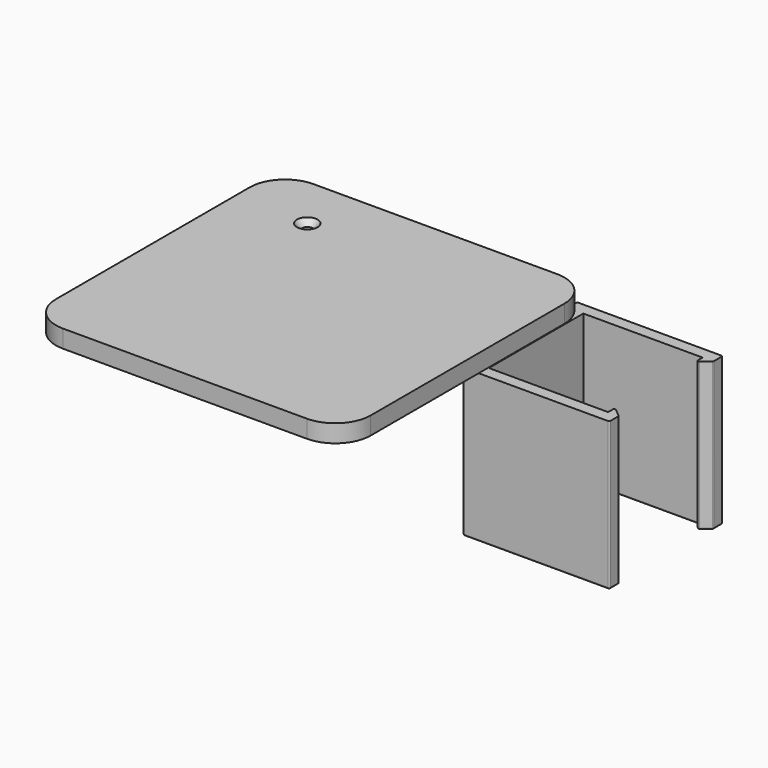
from build123d import *

# Parameters (mm, degrees)
F1_DEPTH          = 2.55
F3_DEPTH          = 22.5
F4_W              = 5
F4_H              = 12.2
F5_DEPTH          = 25
F6_W              = 1.5
F6_H              = 12.3
F7_DEPTH          = 22.5
F8_SIZE2          = 5
F8_SIZE           = 10
F9_W              = 10
F9_H              = 7
F10_DEPTH         = 25
F11_W             = 5
F11_H             = 12.2
F12_DEPTH         = 1.5
F13_R             = 4.5
F14_DEPTH         = 22.5
F17_DEPTH         = 3
F19_D             = 1.778
F19_DEPTH         = 12
F19_CSINK_D       = 3.5052
F19_CSINK_ANGLE   = 82
F19_TIP           = 0.5341650903
F19_2_D           = 1.778
F19_2_DEPTH       = 12
F19_2_CSINK_D     = 3.5052
F19_2_CSINK_ANGLE = 82
F19_2_TIP         = 0.5341650903
F20_W             = 2
F20_H             = 25.05
F21_DEPTH         = 22
F22_W             = 2
F22_H             = 25.05
F23_DEPTH         = 6
F25_DEPTH         = 25.05
F26_R             = 0.25
F27_R             = 0.25
F28_R             = 0.25
F29_R             = 0.25
F30_W             = 6
F30_H             = 0.5
F30_H_2           = 1
F31_DEPTH         = 40
F33_DEPTH         = 25.051
F35_DEPTH         = 25.05
F36_R             = 0.24999


# Not quite as in the source:
# - a fillet or chamfer is up to 0.001 mm smaller than in the source, because OpenCascade refuses the exact size


with BuildPart() as f1:
    # F0 (on Top) → F1 (new body)
    with BuildSketch(Plane.XY):
        with BuildLine():
            ThreePointArc((26.65, 20.5), (24.8926406871, 24.7426406871), (20.65, 26.5))
            Line((20.65, 26.5), (-20.65, 26.5))
            ThreePointArc((-20.65, 26.5), (-24.8926406871, 24.7426406871), (-26.65, 20.5))
            Line((-26.65, 20.5), (-26.65, -20.5))
            ThreePointArc((-26.65, -20.5), (-24.8926406871, -24.7426406871), (-20.65, -26.5))
            Line((-20.65, -26.5), (20.65, -26.5))
            ThreePointArc((20.65, -26.5), (24.8926406871, -24.7426406871), (26.65, -20.5))
            Line((26.65, -20.5), (26.65, 20.5))
        make_face()
    extrude(amount=F1_DEPTH)

    # F2 (on face) → F3 (join)
    with BuildSketch(Plane.XY.offset(2.55)):
        with BuildLine():
            Line((26.65, -20.5), (26.65, 20.5))
            ThreePointArc((26.65, 20.5), (24.8926406871, 24.7426406871), (20.65, 26.5))
            Line((20.65, 26.5), (-20.65, 26.5))
            ThreePointArc((-20.65, 26.5), (-24.8926406871, 24.7426406871), (-26.65, 20.5))
            Line((-26.65, 20.5), (-26.65, -20.5))
            ThreePointArc((-26.65, -20.5), (-24.8926406871, -24.7426406871), (-20.65, -26.5))
            Line((-20.65, -26.5), (20.65, -26.5))
            ThreePointArc((20.65, -26.5), (24.8926406871, -24.7426406871), (26.65, -20.5))
        make_face()
        with BuildLine():
            Line((-20, 24), (20, 24))
            ThreePointArc((20, 24), (22.8284271247, 22.8284271247), (24, 20))
            Line((24, 20), (24, -20))
            ThreePointArc((24, -20), (22.8284271247, -22.8284271247), (20, -24))
            Line((20, -24), (-20, -24))
            ThreePointArc((-20, -24), (-22.8284271247, -22.8284271247), (-24, -20))
            Line((-24, -20), (-24, 20))
            ThreePointArc((-24, 20), (-22.8284271247, 22.8284271247), (-20, 24))
        make_face(mode=Mode.SUBTRACT)
    extrude(amount=F3_DEPTH)

    # F4 (on face) → F5 (cut)
    with BuildSketch(Plane.XZ.offset(26.5)):
        with Locations((-13, 14.45)):
            Rectangle(F4_W, F4_H)
        with Locations((0.5, 14.45)):
            Rectangle(F4_W, F4_H)
    extrude(amount=-F5_DEPTH, mode=Mode.SUBTRACT)

    # F6 (on face) → F7 (join, through all)
    with BuildSketch(Plane.XY.offset(2.55)):
        with Locations((2.25, 17.85)):
            Rectangle(F6_W, F6_H)
    extrude(amount=F7_DEPTH)

    # F8
    f8_edges = [f1.edges().sort_by_distance(p)[0] for p in [
        (2.25, 11.7, 25.05),
    ]]
    f8_side = f1.faces().sort_by_distance((2.25, 11.7, 13.8))[0]
    chamfer(f8_edges, length=F8_SIZE, length2=F8_SIZE2, reference=f8_side)

    # F9 (on face) → F10 (cut)
    with BuildSketch(Plane.XZ.offset(-24)):
        with Locations((9, 6.05)):
            Rectangle(F9_W, F9_H)
    extrude(amount=-F10_DEPTH, mode=Mode.SUBTRACT)

    # F11 (on face) → F12 (cut)
    with BuildSketch(Plane(origin=(0, -24, 0), x_dir=(-1, 0, 0), z_dir=(0, 1, 0))):
        with Locations((-0.5, 14.45)):
            Rectangle(F11_W, F11_H)
        with Locations((13, 14.45)):
            Rectangle(F11_W, F11_H)
    extrude(amount=-F12_DEPTH, mode=Mode.SUBTRACT)

    # F13 (on face) → F14 (join, through all)
    with BuildSketch(Plane.XY.offset(2.55)):
        with Locations((-14.2497913912, 17.2)):
            Circle(F13_R)
    extrude(amount=F14_DEPTH)

    # F19
    with Locations(Plane.XY.offset(28.15)):
        with Locations((-14.2497913912, 17.2)):
            CounterSinkHole(F19_D / 2, F19_CSINK_D / 2, depth=F19_DEPTH, counter_sink_angle=F19_CSINK_ANGLE)
            with Locations((0, 0, -(F19_DEPTH + F19_TIP / 2))):  # 118° drill point
                Cone(0, F19_D / 2, F19_TIP, mode=Mode.SUBTRACT)

    # F20 (on face) → F21 (join)
    with BuildSketch(Plane.YZ.offset(26.65)):
        with Locations((3.5, 12.525)):
            Rectangle(F20_W, F20_H)
    extrude(amount=F21_DEPTH)



with BuildPart() as f17:
    # F16 (on offset) → F17 (new body)
    with BuildSketch(Plane.XY.offset(25.15)):
        with BuildLine():
            ThreePointArc((26.65, 20.5), (24.8926406871, 24.7426406871), (20.65, 26.5))
            Line((20.65, 26.5), (-20.65, 26.5))
            ThreePointArc((-20.65, 26.5), (-24.8926406871, 24.7426406871), (-26.65, 20.5))
            Line((-26.65, 20.5), (-26.65, -20.5))
            ThreePointArc((-26.65, -20.5), (-24.8926406871, -24.7426406871), (-20.65, -26.5))
            Line((-20.65, -26.5), (20.65, -26.5))
            ThreePointArc((20.65, -26.5), (24.8926406871, -24.7426406871), (26.65, -20.5))
            Line((26.65, -20.5), (26.65, 20.5))
        make_face()
    extrude(amount=F17_DEPTH)

    # F19#2
    with Locations(Plane.XY.offset(28.15)):
        with Locations((-14.2497913912, 17.2)):
            CounterSinkHole(F19_2_D / 2, F19_2_CSINK_D / 2, depth=F19_2_DEPTH, counter_sink_angle=F19_2_CSINK_ANGLE)
            with Locations((0, 0, -(F19_2_DEPTH + F19_2_TIP / 2))):  # 118° drill point
                Cone(0, F19_2_D / 2, F19_2_TIP, mode=Mode.SUBTRACT)


with BuildPart() as f21:
    # F20 (on face) → F21, piece 2 (new body)
    with BuildSketch(Plane.YZ.offset(26.65)):
        with Locations((25.5, 12.525)):
            Rectangle(F20_W, F20_H)
    extrude(amount=F21_DEPTH)


with BuildPart() as f1_1:
    add(f1.part)

    add(f21.part)  # F23 merges F21
    # F22 (on face) → F23 (join, through all)
    with BuildSketch(Plane(origin=(26.65, 0, 0), x_dir=(0, -1, 0), z_dir=(-1, 0, 0))):
        with Locations((-25.5, 12.525)):
            Rectangle(F22_W, F22_H)
    extrude(amount=F23_DEPTH)

    # F24 (on face) → F25 (join, through all)
    with BuildSketch(Plane.XY.offset(25.05)):
        Polygon((46.85, 23), (48.65, 24.5), (46.85, 24.5), align=None)
        Polygon((46.85, 6), (46.85, 4.5), (48.65, 4.5), align=None)
    extrude(amount=-F25_DEPTH)

    # F26
    f26_edges = [f1_1.edges().sort_by_distance(p)[0] for p in [
        (46.85, 23, 12.525),
        (46.85, 6, 12.525),
    ]]
    fillet(f26_edges, radius=F26_R)

    # F27
    f27_edges = [f1_1.edges().sort_by_distance(p)[0] for p in [
        (48.65, 26.5, 12.525),
        (48.65, 2.5, 12.525),
        (37.65, 2.5, 0),
        (14, 26.5, 0),
        (48.65, 25.5, 0),
        (48.65, 3.5, 0),
        (48.65, 4.5, 12.525),
        (48.65, 24.5, 12.525),
        (47.955023, 23.920853, 0),
        (47.955023, 5.079147, 0),
    ]]
    fillet(f27_edges, radius=F27_R)

    # F28
    f28_edges = [f1_1.edges().sort_by_distance(p)[0] for p in [
        (14, 24, 6.05),
        (14, 26.5, 6.05),
        (9, 26.5, 2.55),
        (4, 26.5, 6.05),
        (4, 24, 6.05),
    ]]
    fillet(f28_edges, radius=F28_R)

    # F29
    f29_edges = [f1_1.edges().sort_by_distance(p)[0] for p in [
        (-2, -26.5, 14.45),
        (-2, -24, 14.45),
        (-10.5, -26.5, 14.45),
        (-15.5, -26.5, 14.45),
        (-15.5, -24, 14.45),
        (-13, -26.5, 8.35),
        (-13, -24, 8.35),
        (0.5, -26.5, 8.35),
        (0.5, -24, 8.35),
        (3, -24, 14.45),
        (3, -26.5, 14.45),
        (-10.5, -24, 14.45),
    ]]
    fillet(f29_edges, radius=F29_R)

    # F30 (on face) → F31 (cut)
    with BuildSketch(Plane.XY.offset(2.55)):
        with BuildLine():
            Line((24, 13.4), (-24, 13.4))
            Line((-24, 13.4), (-24, -20.5))
            ThreePointArc((-24, -20.5), (-22.8284271247, -23.3284271247), (-20, -24.5))
            Line((-20, -24.5), (-16, -24.5))
            Line((-16, -24.5), (-16, -24))
            Line((-16, -24), (-10, -24))
            Line((-10, -24), (-10, -24.5))
            Line((-10, -24.5), (-2.5, -24.5))
            Line((-2.5, -24.5), (-2.5, -24))
            Line((-2.5, -24), (3.5, -24))
            Line((3.5, -24), (3.5, -24.5))
            Line((3.5, -24.5), (20, -24.5))
            ThreePointArc((20, -24.5), (22.8284271247, -23.3284271247), (24, -20.5))
            Line((24, -20.5), (24, 13.4))
        make_face()
        with Locations((-13, -24.25)):
            Rectangle(F30_W, F30_H)
        with Locations((-13, -25)):
            Rectangle(F30_W, F30_H_2)
        with Locations((0.5, -25)):
            Rectangle(F30_W, F30_H_2)
        with Locations((0.5, -24.25)):
            Rectangle(F30_W, F30_H)
    extrude(amount=F31_DEPTH, mode=Mode.SUBTRACT)

    # F32 (on face) → F33 (cut, through all)
    with BuildSketch(Plane.XY.offset(25.05)):
        with BuildLine():
            Line((-26.65, 2.5), (-24, 2.5))
            Line((-24, 2.5), (-24, 20))
            ThreePointArc((-24, 20), (-22.8284271247, 22.8284271247), (-20, 24))
            Line((-20, 24), (1.5, 24))
            Line((1.5, 24), (1.5, 16.7))
            Line((1.5, 16.7), (3, 16.7))
            Line((3, 16.7), (3, 24))
            Line((3, 24), (20, 24))
            ThreePointArc((20, 24), (22.8284271247, 22.8284271247), (24, 20))
            Line((24, 20), (24, 26.5))
            Line((24, 26.5), (-20.65, 26.5))
            ThreePointArc((-20.65, 26.5), (-24.8926406871, 24.7426406871), (-26.65, 20.5))
            Line((-26.65, 20.5), (-26.65, 2.5))
        make_face()
        with BuildLine():
            Line((26.65, -30.1466379315), (26.65, -20.5))
            ThreePointArc((26.65, -20.5), (24.8926406871, -24.7426406871), (20.65, -26.5))
            Line((20.65, -26.5), (-20.65, -26.5))
            ThreePointArc((-20.65, -26.5), (-24.8926406871, -24.7426406871), (-26.65, -20.5))
            Line((-26.65, -20.5), (-26.65, 2.5))
            Line((-26.65, 2.5), (-34.1783799231, 2.5))
            Line((-34.1783799231, 2.5), (-34.1783799231, -30.1466379315))
            Line((-34.1783799231, -30.1466379315), (26.65, -30.1466379315))
        make_face()
        with BuildLine():
            Line((-34.1783799231, 2.5), (-26.65, 2.5))
            Line((-26.65, 2.5), (-26.65, 20.5))
            ThreePointArc((-26.65, 20.5), (-24.8926406871, 24.7426406871), (-20.65, 26.5))
            Line((-20.65, 26.5), (24, 26.5))
            Line((24, 26.5), (24, 32.8557267785))
            Line((24, 32.8557267785), (-34.1783799231, 32.8557267785))
            Line((-34.1783799231, 32.8557267785), (-34.1783799231, 2.5))
        make_face()
        with BuildLine():
            Line((-24, 2.5), (24, 2.5))
            Line((24, 2.5), (24, 20))
            ThreePointArc((24, 20), (22.8284271247, 22.8284271247), (20, 24))
            Line((20, 24), (3, 24))
            Line((3, 24), (3, 16.7))
            Line((3, 16.7), (1.5, 16.7))
            Line((1.5, 16.7), (1.5, 24))
            Line((1.5, 24), (-20, 24))
            ThreePointArc((-20, 24), (-22.8284271247, 22.8284271247), (-24, 20))
            Line((-24, 20), (-24, 2.5))
        make_face()
        with BuildLine():
            Line((26.65, -20.5), (26.65, 2.5))
            Line((26.65, 2.5), (24, 2.5))
            Line((24, 2.5), (24, -20.5))
            ThreePointArc((24, -20.5), (22.8284271247, -23.3284271247), (20, -24.5))
            Line((20, -24.5), (3.5, -24.5))
            Line((3.5, -24.5), (3.5, -25.5))
            Line((3.5, -25.5), (-2.5, -25.5))
            Line((-2.5, -25.5), (-2.5, -24.5))
            Line((-2.5, -24.5), (-10, -24.5))
            Line((-10, -24.5), (-10, -25.5))
            Line((-10, -25.5), (-16, -25.5))
            Line((-16, -25.5), (-16, -24.5))
            Line((-16, -24.5), (-20, -24.5))
            ThreePointArc((-20, -24.5), (-22.8284271247, -23.3284271247), (-24, -20.5))
            Line((-24, -20.5), (-24, 2.5))
            Line((-24, 2.5), (-26.65, 2.5))
            Line((-26.65, 2.5), (-26.65, -20.5))
            ThreePointArc((-26.65, -20.5), (-24.8926406871, -24.7426406871), (-20.65, -26.5))
            Line((-20.65, -26.5), (20.65, -26.5))
            ThreePointArc((20.65, -26.5), (24.8926406871, -24.7426406871), (26.65, -20.5))
        make_face()
        with BuildLine():
            Line((24, -20.5), (24, 2.5))
            Line((24, 2.5), (-24, 2.5))
            Line((-24, 2.5), (-24, -20.5))
            ThreePointArc((-24, -20.5), (-22.8284271247, -23.3284271247), (-20, -24.5))
            Line((-20, -24.5), (-16, -24.5))
            Line((-16, -24.5), (-16, -25.5))
            Line((-16, -25.5), (-10, -25.5))
            Line((-10, -25.5), (-10, -24.5))
            Line((-10, -24.5), (-2.5, -24.5))
            Line((-2.5, -24.5), (-2.5, -25.5))
            Line((-2.5, -25.5), (3.5, -25.5))
            Line((3.5, -25.5), (3.5, -24.5))
            Line((3.5, -24.5), (20, -24.5))
            ThreePointArc((20, -24.5), (22.8284271247, -23.3284271247), (24, -20.5))
        make_face()
    extrude(amount=-F33_DEPTH, mode=Mode.SUBTRACT)

    # F34 (on face) → F35 (join, through all)
    with BuildSketch(Plane.XY.offset(25.05)):
        with BuildLine():
            Line((24, 20.5), (26.65, 20.5))
            ThreePointArc((26.65, 20.5), (26.2550341538, 22.6409325386), (25.122135955, 24.5))
            Line((25.122135955, 24.5), (26.65, 24.5))
            Line((26.65, 24.5), (26.65, 25.159496814))
            Line((26.65, 25.159496814), (24, 25.159496814))
            Line((24, 25.159496814), (24, 20.5))
        make_face()
        with BuildLine():
            ThreePointArc((25.122135955, 24.5), (26.2550341538, 22.6409325386), (26.65, 20.5))
            Line((26.65, 20.5), (26.65, 24.5))
            Line((26.65, 24.5), (25.122135955, 24.5))
        make_face()
    extrude(amount=-F35_DEPTH)

    # F36 (radius 0.25 in the source; OpenCascade refuses exactly that, so slightly less here)
    f36_edges = [f1_1.edges().sort_by_distance(p)[0] for p in [
        (26.65, 14.5, 0),
        (36.875, 24.5, 0),
        (36.875, 4.5, 0),
        (25.2, 2.5, 0),
        (24, 14.375, 0),
        (24, 26.426777, 0.073223),
        (24, 26.5, 12.65),
    ]]
    fillet(f36_edges, radius=F36_R)


solid = Compound([f17.part, f1_1.part])
